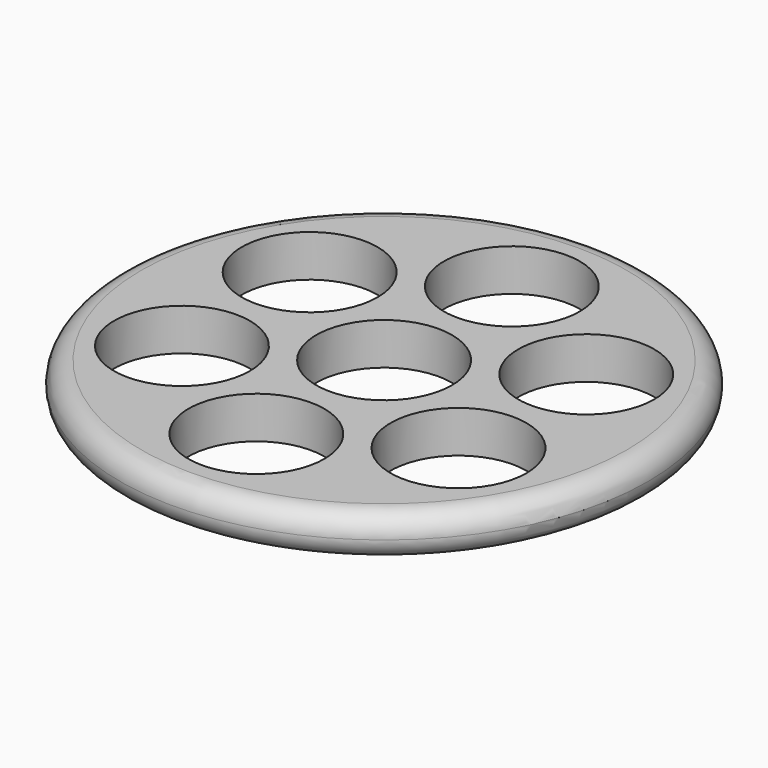
from build123d import *

# Parameters (mm, degrees)
F0_R     = 44
F0_R_2   = 11.325
F1_DEPTH = 7
F2_R     = 3.5
F3_R     = 3.49999


# Not quite as in the source:
# - a fillet or chamfer is up to 0.001 mm smaller than in the source, because OpenCascade refuses the exact size


with BuildPart() as f1:
    # F0 (on Top) → F1 (new body)
    with BuildSketch(Plane.XY):
        Circle(F0_R)
        with Locations((-23.0534838522, -13.3099351078)):
            Circle(F0_R_2, mode=Mode.SUBTRACT)
        with Locations((0, -26.6198702157)):
            Circle(F0_R_2, mode=Mode.SUBTRACT)
        with Locations((23.0534838522, -13.3099351078)):
            Circle(F0_R_2, mode=Mode.SUBTRACT)
        with Locations((-23.0534838522, 13.3099351078)):
            Circle(F0_R_2, mode=Mode.SUBTRACT)
        Circle(F0_R_2, mode=Mode.SUBTRACT)
        with Locations((23.0534838522, 13.3099351078)):
            Circle(F0_R_2, mode=Mode.SUBTRACT)
        with Locations((0, 26.6198702157)):
            Circle(F0_R_2, mode=Mode.SUBTRACT)
    extrude(amount=F1_DEPTH)

    # F2
    f2_edges = [f1.edges().sort_by_distance(p)[0] for p in [
        (-44, 0, 7),
    ]]
    fillet(f2_edges, radius=F2_R)

    # F3 (radius 3.5 in the source; OpenCascade refuses exactly that, so slightly less here)
    f3_edges = [f1.edges().sort_by_distance(p)[0] for p in [
        (-44, 0, 0),
    ]]
    fillet(f3_edges, radius=F3_R)


solid = f1.part
